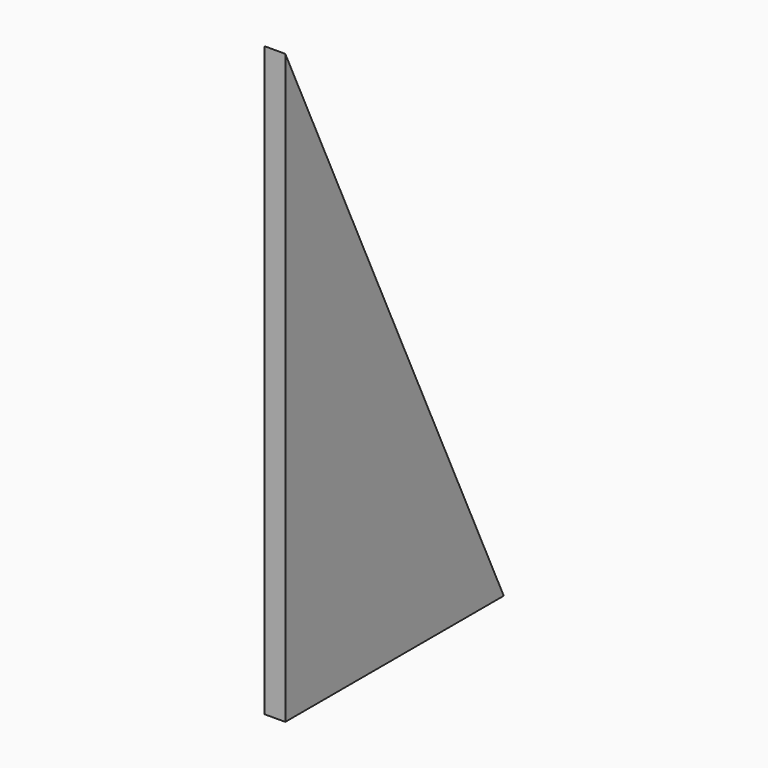
from build123d import *

# Parameters (mm, degrees)
F2_DEPTH = 12.7


# Not quite as in the source:
# - a variable given as a bare number and used for a length is read in inches; the dataset says mm whatever the document's units were


with BuildPart() as f2:
    # F1 (on Right) → F2 (new body)
    with BuildSketch(Plane.YZ):
        Polygon((0, 351.5985079486), (0, -4.0014920514), (165.1, -4.0014920514), align=None)
    extrude(amount=F2_DEPTH)


solid = f2.part
